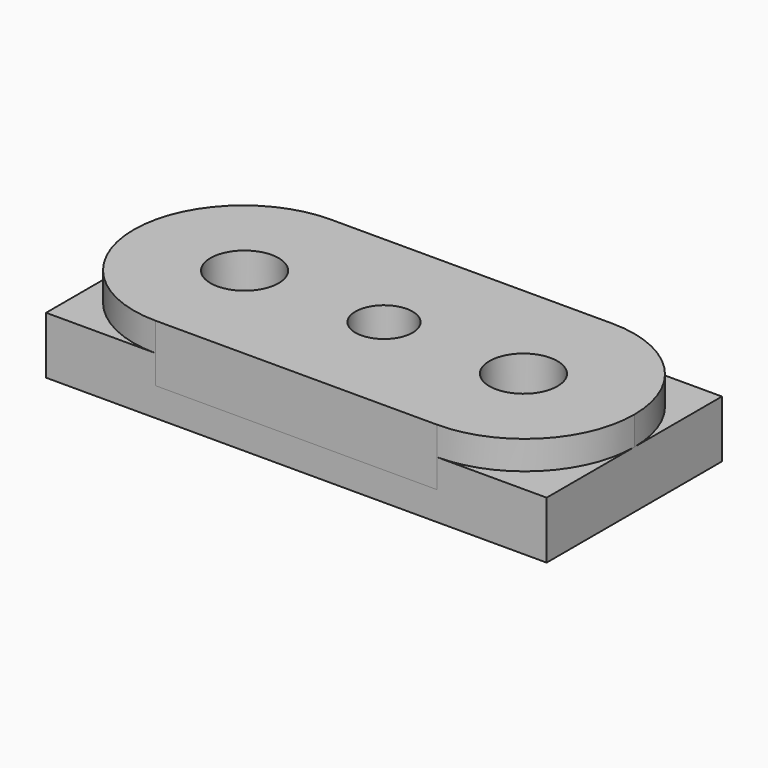
from build123d import *

# Parameters (mm, degrees)
F0_W     = 70
F0_H     = 30.6375
F0_R     = 10.31875
F1_DEPTH = 4
F2_DEPTH = 8
F3_D     = 9.525
F4_D     = 8
F5_R     = 15.31874


# Not quite as in the source:
# - a fillet or chamfer is up to 0.001 mm smaller than in the source, because OpenCascade refuses the exact size
# - a length typed as a fraction of an inch, garbled in the dataset ("3 / 203.2 mm" for 3/8 in), is restored


with BuildPart() as f1:
    # F0 (on Top) → F1 (new body, symmetric)
    with BuildSketch(Plane.XY):
        Rectangle(F0_W, F0_H)
        with Locations((-19.5, 0)):
            Circle(F0_R, mode=Mode.SUBTRACT)
        with BuildLine():
            Line((4.05, 4), (4.05, 0))
            Line((4.05, 0), (4.05, -4))
            ThreePointArc((4.05, -4), (0, -8.05), (-4.05, -4))
            Line((-4.05, -4), (-4.05, 0))
            Line((-4.05, 0), (-4.05, 4))
            ThreePointArc((-4.05, 4), (0, 8.05), (4.05, 4))
        make_face(mode=Mode.SUBTRACT)
        with Locations((19.5, 0)):
            Circle(F0_R, mode=Mode.SUBTRACT)
    extrude(amount=F1_DEPTH, both=True)


with BuildPart() as f2:
    # F0 (on Top) → F2 (new body)
    with BuildSketch(Plane.XY):
        Rectangle(F0_W, F0_H)
        with Locations((-19.5, 0)):
            Circle(F0_R, mode=Mode.SUBTRACT)
        with BuildLine():
            Line((4.05, 4), (4.05, 0))
            Line((4.05, 0), (4.05, -4))
            ThreePointArc((4.05, -4), (0, -8.05), (-4.05, -4))
            Line((-4.05, -4), (-4.05, 0))
            Line((-4.05, 0), (-4.05, 4))
            ThreePointArc((-4.05, 4), (0, 8.05), (4.05, 4))
        make_face(mode=Mode.SUBTRACT)
        with Locations((19.5, 0)):
            Circle(F0_R, mode=Mode.SUBTRACT)
        with Locations((-19.5, 0)):
            Circle(F0_R)
        with BuildLine():
            Line((4.05, -4), (4.05, 0))
            ThreePointArc((4.05, 0), (0, -4.05), (-4.05, 0))
            Line((-4.05, 0), (-4.05, -4))
            ThreePointArc((-4.05, -4), (0, -8.05), (4.05, -4))
        make_face()
        with BuildLine():
            ThreePointArc((-4.05, 0), (0, -4.05), (4.05, 0))
            ThreePointArc((4.05, 0), (0, 4.05), (-4.05, 0))
        make_face()
        with BuildLine():
            ThreePointArc((-4.05, 0), (0, 4.05), (4.05, 0))
            Line((4.05, 0), (4.05, 4))
            ThreePointArc((4.05, 4), (0, 8.05), (-4.05, 4))
            Line((-4.05, 4), (-4.05, 0))
        make_face()
        with Locations((19.5, 0)):
            Circle(F0_R)
    extrude(amount=F2_DEPTH)

    # F3 (through all)
    with Locations(Plane(origin=(0, 0, 0), x_dir=(1, 0, 0), z_dir=(0, 0, -1))):
        with Locations((-19.5, 0), (19.5, 0)):
            Hole(F3_D / 2)

    # F4 (through all)
    with Locations(Plane(origin=(0, 0, 0), x_dir=(1, 0, 0), z_dir=(0, 0, -1))):
        with Locations((0, 0)):
            Hole(F4_D / 2)

    # F5 (radius 15.31875 in the source; OpenCascade refuses exactly that, so slightly less here)
    f5_edges = [f2.edges().sort_by_distance(p)[0] for p in [
        (-35, 15.31875, 4),
        (35, 15.31875, 4),
        (-35, -15.31875, 4),
        (35, -15.31875, 4),
    ]]
    fillet(f5_edges, radius=F5_R)


solid = Compound([f1.part, f2.part])
